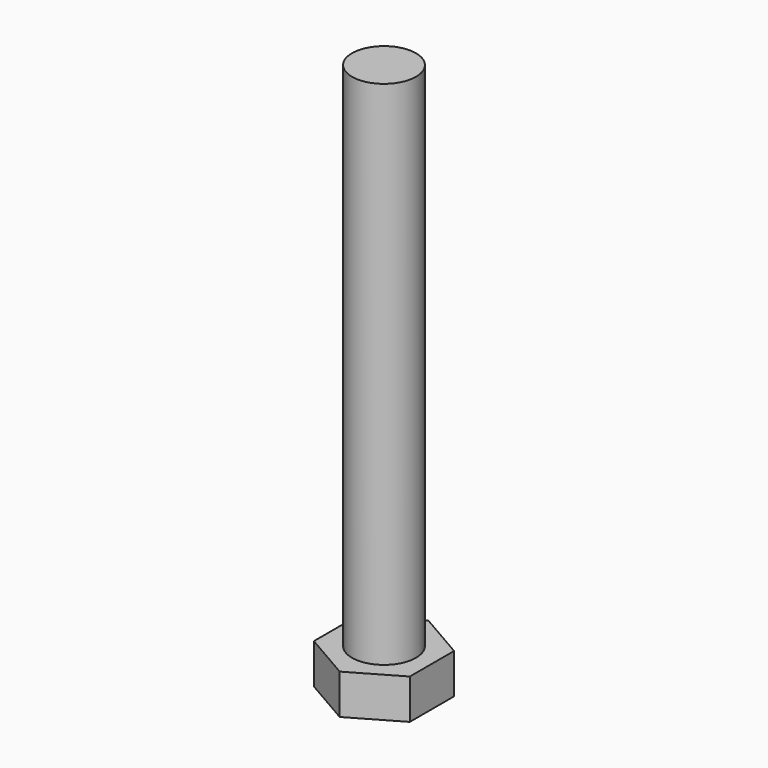
from build123d import *

# Parameters (mm, degrees)
F1_R     = 6.35
F2_DEPTH = 7.9375
F3_DEPTH = 109.5375


# Not quite as in the source:
# - a variable given as a bare number and used for a length is read in inches; the dataset says mm whatever the document's units were


with BuildPart() as f2:
    # F1 (on Top) → F2 (new body)
    with BuildSketch(Plane.XY):
        Polygon((9.525, -5.499261314), (9.525, 5.499261314), (0, 10.9985226281), (-9.525, 5.499261314), (-9.525, -5.499261314), (0, -10.9985226281), align=None)
        Circle(F1_R, mode=Mode.SUBTRACT)
    extrude(amount=F2_DEPTH)

    # F1 (on Top) → F3 (join)
    with BuildSketch(Plane.XY):
        Circle(F1_R)
    extrude(amount=F3_DEPTH)


solid = f2.part
